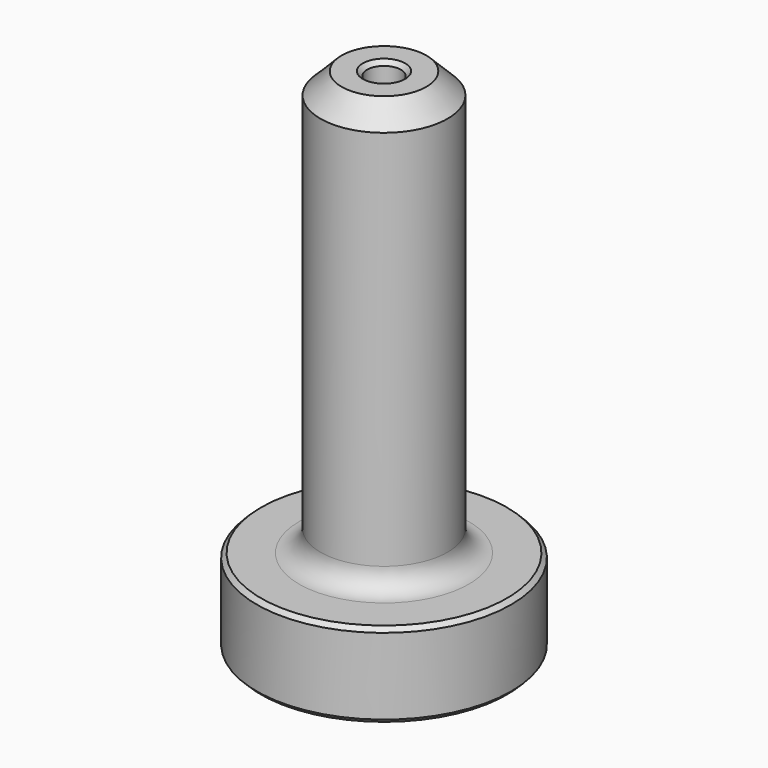
from build123d import *

# Parameters (mm, degrees)
F2_SIZE        = 5
F3_SIZE        = 0.99999
F5_R           = 5
F6_D           = 10.3
F6_DEPTH       = 35.25
F6_TIP         = 3.094432188
F8_D           = 8
F8_DEPTH       = 15
F8_CSINK_D     = 10
F8_CSINK_ANGLE = 90
F8_TIP         = 2.4034424761


# Not quite as in the source:
# - a fillet or chamfer is up to 0.001 mm smaller than in the source, because OpenCascade refuses the exact size


with BuildPart() as f1:
    # F0 (on Front) → F1 (revolve)
    with BuildSketch(Plane.XZ):
        Polygon((-27, 0), (0, 0), (0, 118), (-15, 118), (-15, 18), (-30, 18), (-30, -2), (-27, -2), align=None)
    revolve(axis=Axis((0, 0, 59), (0, 0, -1)))

    # F2
    f2_edges = [f1.edges().sort_by_distance(p)[0] for p in [
        (15, 0, 118),
    ]]
    chamfer(f2_edges, length=F2_SIZE)

    # F3 (size 1 in the source; OpenCascade refuses exactly that, so slightly less here)
    f3_edges = [f1.edges().sort_by_distance(p)[0] for p in [
        (30, 0, 18),
        (30, 0, -2),
        (27, 0, -2),
        (27, 0, 0),
        (-27, 0, -1),
    ]]
    chamfer(f3_edges, length=F3_SIZE)

    # F5
    f5_edges = [f1.edges().sort_by_distance(p)[0] for p in [
        (15, 0, 18),
    ]]
    fillet(f5_edges, radius=F5_R)

    # F6
    with Locations(Plane(origin=(0, 0, 0), x_dir=(1, 0, 0), z_dir=(0, 0, -1))):
        with Locations((0, 0)):
            Hole(F6_D / 2, depth=F6_DEPTH)
            with Locations((0, 0, -(F6_DEPTH + F6_TIP / 2))):  # 118° drill point
                Cone(0, F6_D / 2, F6_TIP, mode=Mode.SUBTRACT)

    # F8
    with Locations(Plane.XY.offset(118)):
        with Locations((0, 0)):
            CounterSinkHole(F8_D / 2, F8_CSINK_D / 2, depth=F8_DEPTH, counter_sink_angle=F8_CSINK_ANGLE)
            with Locations((0, 0, -(F8_DEPTH + F8_TIP / 2))):  # 118° drill point
                Cone(0, F8_D / 2, F8_TIP, mode=Mode.SUBTRACT)


solid = f1.part
